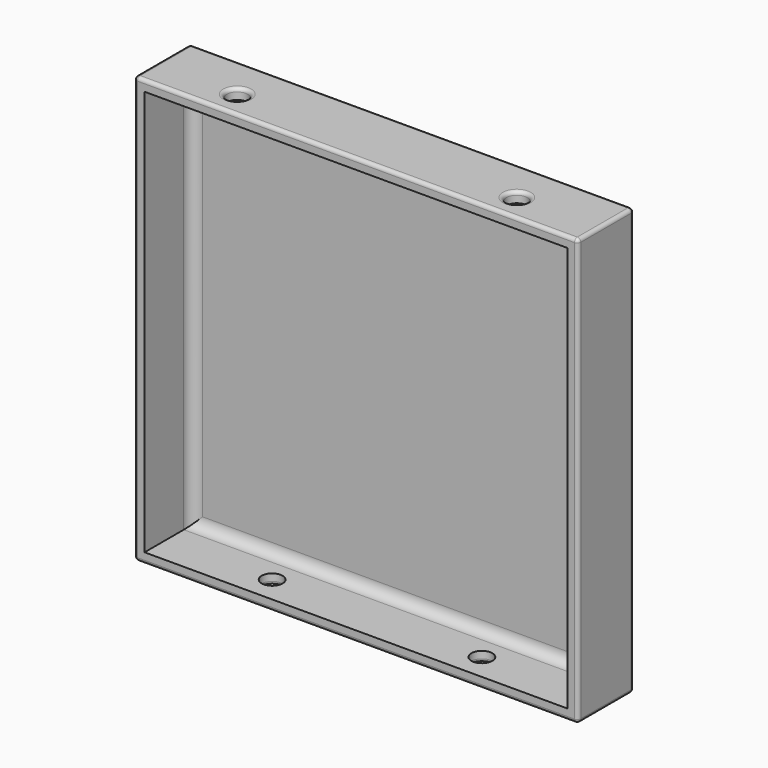
from build123d import *

# Parameters (mm, degrees)
F0_W     = 127
F0_H     = 122
F1_DEPTH = 20
F2_T     = -3
F4_D     = 6
F4_DEPTH = 3.001
F6_D     = 6
F6_DEPTH = 3.001
F7_R     = 3
F9_DEPTH = 2
F10_R    = 1


# Not quite as in the source:
# - ends of sketch curves that miss each other by under 0.0002 mm in the source are joined


with BuildPart() as f1:
    # F0 (on Front) → F1 (new body)
    with BuildSketch(Plane.XZ):
        Rectangle(F0_W, F0_H)
    extrude(amount=F1_DEPTH)

    # F2
    f2_openings = [f1.faces().sort_by_distance(p)[0] for p in [
        (0, -20, 0),
    ]]
    offset(amount=F2_T, openings=f2_openings)

    # F4 (through all, one way)
    with BuildSketch(Plane(origin=(0, 0, 58), x_dir=(1, 0, 0), z_dir=(0, 0, -1))):
        with Locations((-40, 12.5), (40, 12.5)):
            Circle(F4_D / 2)
    extrude(amount=-F4_DEPTH, mode=Mode.SUBTRACT)

    # F6 (through all, one way)
    with BuildSketch(Plane.XY.offset(-58)):
        with Locations((-30, -12.5), (30, -12.5)):
            Circle(F6_D / 2)
    extrude(amount=-F6_DEPTH, mode=Mode.SUBTRACT)

    # F7
    f7_edges = [f1.edges().sort_by_distance(p)[0] for p in [
        (0, -3, 58),
        (-60.5, -3, 0),
        (0, -3, -58),
        (60.5, -3, 0),
    ]]
    fillet(f7_edges, radius=F7_R)

    # F8 (on face) → F9 (cut)
    with BuildSketch(Plane(origin=(0, 0, 0), x_dir=(-1, 0, 0), z_dir=(0, 1, 0))):
        with BuildLine():
            Line((-36.955256, 4.469993), (-36.955256, -1.695514))
            add(Edge.make_bspline(
                [(-35.567857, -4.963227), (-36.492789, -4.058952), (-36.955255, -2.969713), (-36.955256, -1.695514)],
                knots=[0, 0, 0, 0, 1, 1, 1, 1], degree=3))
            add(Edge.make_bspline(
                [(-32.225487, -6.319638), (-33.528801, -6.319638), (-34.642924, -5.867501), (-35.567857, -4.963227)],
                knots=[0, 0, 0, 0, 1, 1, 1, 1], degree=3))
            Line((-32.225487, -6.319638), (-29.072308, -6.319638))
            add(Edge.make_bspline(
                [(-25.729939, -4.963227), (-26.654871, -5.867501), (-27.768995, -6.319638), (-29.072308, -6.319638)],
                knots=[0, 0, 0, 0, 1, 1, 1, 1], degree=3))
            add(Edge.make_bspline(
                [(-25.682643, -4.916993), (-25.703662, -4.937556), (-25.719427, -4.952967), (-25.729939, -4.963227)],
                knots=[0, 0, 0, 0, 1, 1, 1, 1], degree=3))
            Line((-25.682643, -4.916993), (-22.765952, -6.62792))
            Line((-22.765952, -6.62792), (-22.765952, 9.094123))
            Line((-22.765952, 9.094123), (-25.919131, 9.094123))
            Line((-25.919131, 9.094123), (-25.919131, 7.907261))
            add(Edge.make_bspline(
                [(-29.07231, 9.094123), (-27.853081, 9.094123), (-26.802021, 8.698503), (-25.919131, 7.907261)],
                knots=[0, 0, 0, 0, 1, 1, 1, 1], degree=3))
            Line((-29.07231, 9.094123), (-32.225488, 9.094123))
            add(Edge.make_bspline(
                [(-35.567858, 7.737712), (-34.642925, 8.641986), (-33.528802, 9.094123), (-32.225488, 9.094123)],
                knots=[0, 0, 0, 0, 1, 1, 1, 1], degree=3))
            add(Edge.make_bspline(
                [(-36.955256, 4.469993), (-36.955256, 5.744198), (-36.49279, 6.833437), (-35.567858, 7.737712)],
                knots=[0, 0, 0, 0, 1, 1, 1, 1], degree=3))
        make_face()
        with BuildLine():
            Line((-33.802078, -1.695514), (-33.802078, 4.469993))
            add(Edge.make_bspline(
                [(-33.344867, 5.54896), (-33.649674, 5.250959), (-33.802078, 4.891304), (-33.802078, 4.469993)],
                knots=[0, 0, 0, 0, 1, 1, 1, 1], degree=3))
            add(Edge.make_bspline(
                [(-32.225488, 6.01137), (-32.656423, 6.01137), (-33.029549, 5.857233), (-33.344867, 5.54896)],
                knots=[0, 0, 0, 0, 1, 1, 1, 1], degree=3))
            Line((-32.225488, 6.01137), (-29.07231, 6.01137))
            add(Edge.make_bspline(
                [(-27.180403, 5.54896), (-28.01074, 5.857233), (-28.641376, 6.01137), (-29.07231, 6.01137)],
                knots=[0, 0, 0, 0, 1, 1, 1, 1], degree=3))
            add(Edge.make_bspline(
                [(-25.919131, 4.469993), (-25.919131, 4.891304), (-26.339555, 5.250959), (-27.180403, 5.54896)],
                knots=[0, 0, 0, 0, 1, 1, 1, 1], degree=3))
            Line((-25.919131, 4.469993), (-25.919131, -1.695514))
            add(Edge.make_bspline(
                [(-27.180403, -2.78989), (-26.339555, -2.481617), (-25.919131, -2.116825), (-25.919131, -1.695514)],
                knots=[0, 0, 0, 0, 1, 1, 1, 1], degree=3))
            add(Edge.make_bspline(
                [(-29.07231, -3.236891), (-28.641376, -3.236891), (-28.01074, -3.087891), (-27.180403, -2.78989)],
                knots=[0, 0, 0, 0, 1, 1, 1, 1], degree=3))
            Line((-29.07231, -3.236891), (-32.225488, -3.236891))
            add(Edge.make_bspline(
                [(-33.344867, -2.78989), (-33.029549, -3.087891), (-32.656423, -3.236891), (-32.225488, -3.236891)],
                knots=[0, 0, 0, 0, 1, 1, 1, 1], degree=3))
            add(Edge.make_bspline(
                [(-33.802078, -1.695514), (-33.802078, -2.116825), (-33.649674, -2.481617), (-33.344867, -2.78989)],
                knots=[0, 0, 0, 0, 1, 1, 1, 1], degree=3))
        make_face(mode=Mode.SUBTRACT)
        with BuildLine():
            add(Edge.make_bspline(
                [(-11.414509, 9.094123), (-10.111195, 9.094123), (-8.997071, 8.641986), (-8.072137, 7.737712)],
                knots=[0, 0, 0, 0, 1, 1, 1, 1], degree=3))
            Line((-11.414509, 9.094123), (-16.144277, 9.094123))
            add(Edge.make_bspline(
                [(-19.486647, 7.737712), (-18.561714, 8.641986), (-17.447591, 9.094123), (-16.144277, 9.094123)],
                knots=[0, 0, 0, 0, 1, 1, 1, 1], degree=3))
            add(Edge.make_bspline(
                [(-20.874045, 4.469993), (-20.874045, 5.744198), (-20.411579, 6.833437), (-19.486647, 7.737712)],
                knots=[0, 0, 0, 0, 1, 1, 1, 1], degree=3))
            Line((-20.874045, 4.469993), (-20.874045, -1.695514))
            add(Edge.make_bspline(
                [(-19.486647, -4.963233), (-20.411579, -4.058959), (-20.874045, -2.969719), (-20.874045, -1.695514)],
                knots=[0, 0, 0, 0, 1, 1, 1, 1], degree=3))
            add(Edge.make_bspline(
                [(-16.144277, -6.319645), (-17.447591, -6.319645), (-18.561714, -5.867508), (-19.486647, -4.963233)],
                knots=[0, 0, 0, 0, 1, 1, 1, 1], degree=3))
            Line((-16.144277, -6.319645), (-11.414509, -6.319645))
            add(Edge.make_bspline(
                [(-8.072137, -4.963233), (-8.997071, -5.867508), (-10.111195, -6.319645), (-11.414509, -6.319645)],
                knots=[0, 0, 0, 0, 1, 1, 1, 1], degree=3))
            add(Edge.make_bspline(
                [(-6.684738, -1.695514), (-6.684738, -2.969719), (-7.147205, -4.058959), (-8.072137, -4.963233)],
                knots=[0, 0, 0, 0, 1, 1, 1, 1], degree=3))
            Line((-6.684738, -1.695514), (-9.83792, -1.695514))
            add(Edge.make_bspline(
                [(-10.310897, -2.78989), (-9.995579, -2.481617), (-9.83792, -2.116825), (-9.83792, -1.695514)],
                knots=[0, 0, 0, 0, 1, 1, 1, 1], degree=3))
            add(Edge.make_bspline(
                [(-11.414509, -3.236891), (-10.983575, -3.236891), (-10.615704, -3.087891), (-10.310897, -2.78989)],
                knots=[0, 0, 0, 0, 1, 1, 1, 1], degree=3))
            Line((-11.414509, -3.236891), (-16.144277, -3.236891))
            add(Edge.make_bspline(
                [(-17.263656, -2.78989), (-16.948338, -3.087891), (-16.575212, -3.236891), (-16.144277, -3.236891)],
                knots=[0, 0, 0, 0, 1, 1, 1, 1], degree=3))
            add(Edge.make_bspline(
                [(-17.720866, -1.695514), (-17.720866, -2.116825), (-17.568463, -2.481617), (-17.263656, -2.78989)],
                knots=[0, 0, 0, 0, 1, 1, 1, 1], degree=3))
            Line((-17.720866, -1.695514), (-17.720866, 4.469993))
            add(Edge.make_bspline(
                [(-17.263656, 5.54896), (-17.568463, 5.250959), (-17.720866, 4.891304), (-17.720866, 4.469993)],
                knots=[0, 0, 0, 0, 1, 1, 1, 1], degree=3))
            add(Edge.make_bspline(
                [(-16.144277, 6.01137), (-16.575212, 6.01137), (-16.948338, 5.857233), (-17.263656, 5.54896)],
                knots=[0, 0, 0, 0, 1, 1, 1, 1], degree=3))
            Line((-16.144277, 6.01137), (-11.414509, 6.01137))
            add(Edge.make_bspline(
                [(-10.310897, 5.54896), (-10.615704, 5.857233), (-10.983575, 6.01137), (-11.414509, 6.01137)],
                knots=[0, 0, 0, 0, 1, 1, 1, 1], degree=3))
            add(Edge.make_bspline(
                [(-9.83792, 4.469993), (-9.83792, 4.891304), (-9.995579, 5.250959), (-10.310897, 5.54896)],
                knots=[0, 0, 0, 0, 1, 1, 1, 1], degree=3))
            Line((-9.83792, 4.469993), (-6.684738, 4.469993))
            add(Edge.make_bspline(
                [(-8.072137, 7.737712), (-7.147205, 6.833437), (-6.684738, 5.744198), (-6.684738, 4.469993)],
                knots=[0, 0, 0, 0, 1, 1, 1, 1], degree=3))
        make_face()
        with BuildLine():
            Line((6.259055, -3.236891), (3.105876, -3.236891))
            add(Edge.make_bspline(
                [(1.9865, -2.78989), (2.30182, -3.087891), (2.674945, -3.236891), (3.105876, -3.236891)],
                knots=[0, 0, 0, 0, 1, 1, 1, 1], degree=3))
            add(Edge.make_bspline(
                [(1.529287, -1.695514), (1.529287, -2.116825), (1.681691, -2.481617), (1.9865, -2.78989)],
                knots=[0, 0, 0, 0, 1, 1, 1, 1], degree=3))
            Line((1.529287, -1.695514), (1.529287, 6.01137))
            Line((1.529287, 6.01137), (6.259055, 6.01137))
            Line((6.259055, 6.01137), (6.259055, 9.094123))
            Line((6.259055, 9.094123), (1.529287, 9.094123))
            Line((1.529287, 9.094123), (1.529287, 12.485152))
            Line((1.529287, 12.485152), (-5.092388, 6.01137))
            Line((-5.092388, 6.01137), (-1.623892, 6.01137))
            Line((-1.623892, 6.01137), (-1.623892, -1.695514))
            add(Edge.make_bspline(
                [(-0.236493, -4.963233), (-1.161425, -4.058959), (-1.623892, -2.969719), (-1.623892, -1.695514)],
                knots=[0, 0, 0, 0, 1, 1, 1, 1], degree=3))
            add(Edge.make_bspline(
                [(3.105876, -6.319645), (1.802563, -6.319645), (0.688439, -5.867508), (-0.236493, -4.963233)],
                knots=[0, 0, 0, 0, 1, 1, 1, 1], degree=3))
            Line((3.105876, -6.319645), (6.259055, -6.319645))
            Line((6.259055, -6.319645), (6.259055, -3.236891))
        make_face()
        with BuildLine():
            Line((8.198265, 9.094123), (8.198265, -1.695514))
            add(Edge.make_bspline(
                [(9.585664, -4.963233), (8.660731, -4.058959), (8.198265, -2.969719), (8.198265, -1.695514)],
                knots=[0, 0, 0, 0, 1, 1, 1, 1], degree=3))
            add(Edge.make_bspline(
                [(12.928033, -6.319645), (11.624719, -6.319645), (10.510596, -5.867508), (9.585664, -4.963233)],
                knots=[0, 0, 0, 0, 1, 1, 1, 1], degree=3))
            Line((12.928033, -6.319645), (14.504622, -6.319645))
            add(Edge.make_bspline(
                [(17.657801, -5.132783), (16.774911, -5.924024), (15.723851, -6.319645), (14.504622, -6.319645)],
                knots=[0, 0, 0, 0, 1, 1, 1, 1], degree=3))
            Line((17.657801, -5.132783), (17.657801, -7.861022))
            add(Edge.make_bspline(
                [(17.184821, -8.939982), (17.500141, -8.641986), (17.657801, -8.282332), (17.657801, -7.861022)],
                knots=[0, 0, 0, 0, 1, 1, 1, 1], degree=3))
            add(Edge.make_bspline(
                [(16.081212, -9.402398), (16.512143, -9.402398), (16.880013, -9.24826), (17.184821, -8.939982)],
                knots=[0, 0, 0, 0, 1, 1, 1, 1], degree=3))
            Line((16.081212, -9.402398), (9.774854, -9.402398))
            Line((9.774854, -9.402398), (9.774854, -12.485152))
            Line((9.774854, -12.485152), (16.081212, -12.485152))
            add(Edge.make_bspline(
                [(19.423581, -11.12874), (18.498649, -12.033015), (17.384526, -12.485152), (16.081212, -12.485152)],
                knots=[0, 0, 0, 0, 1, 1, 1, 1], degree=3))
            add(Edge.make_bspline(
                [(20.81098, -7.861022), (20.81098, -9.135226), (20.348514, -10.224466), (19.423581, -11.12874)],
                knots=[0, 0, 0, 0, 1, 1, 1, 1], degree=3))
            Line((20.81098, -7.861022), (20.81098, 9.094123))
            Line((20.81098, 9.094123), (17.657801, 9.094123))
            Line((17.657801, 9.094123), (17.657801, -1.695514))
            add(Edge.make_bspline(
                [(16.39653, -2.78989), (17.237377, -2.481617), (17.657801, -2.116825), (17.657801, -1.695514)],
                knots=[0, 0, 0, 0, 1, 1, 1, 1], degree=3))
            add(Edge.make_bspline(
                [(14.504622, -3.236891), (14.935553, -3.236891), (15.566189, -3.087891), (16.39653, -2.78989)],
                knots=[0, 0, 0, 0, 1, 1, 1, 1], degree=3))
            Line((14.504622, -3.236891), (12.928033, -3.236891))
            add(Edge.make_bspline(
                [(11.80865, -2.78989), (12.12397, -3.087891), (12.497098, -3.236891), (12.928033, -3.236891)],
                knots=[0, 0, 0, 0, 1, 1, 1, 1], degree=3))
            add(Edge.make_bspline(
                [(11.351444, -1.695514), (11.351444, -2.116825), (11.503846, -2.481617), (11.80865, -2.78989)],
                knots=[0, 0, 0, 0, 1, 1, 1, 1], degree=3))
            Line((11.351444, -1.695514), (11.351444, 9.094123))
            Line((11.351444, 9.094123), (8.198265, 9.094123))
        make_face()
        Polygon((22.765951, 9.094123), (27.968692, 1.387239), (22.765951, -6.319645), (26.549765, -6.319645), (29.860599, -1.418063), (33.17144, -6.319645), (36.955255, -6.319645), (31.752506, 1.387239), (36.955255, 9.094123), (33.17144, 9.094123), (29.860599, 4.192548), (26.549765, 9.094123), align=None)
    extrude(amount=-F9_DEPTH, mode=Mode.SUBTRACT)

    # F10
    f10_edges = [f1.edges().sort_by_distance(p)[0] for p in [
        (63.5, -10, -61),
        (63.5, -10, 61),
        (63.5, 0, 0),
        (63.5, -20, 0),
        (0, 0, 61),
        (0, -20, 61),
        (-63.5, -10, 61),
        (37, -12.5, 61),
        (-43, -12.5, 61),
        (-63.5, -10, -61),
        (-63.5, 0, 0),
        (-63.5, -20, 0),
        (0, 0, -61),
        (0, -20, -61),
        (-33, -12.5, -61),
        (27, -12.5, -61),
    ]]
    fillet(f10_edges, radius=F10_R)


solid = f1.part
